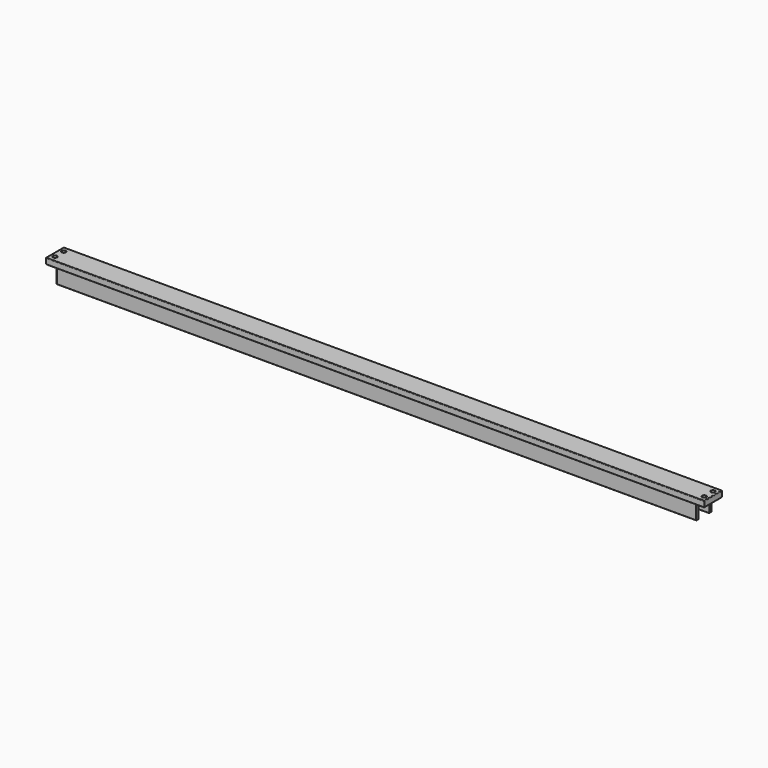
from build123d import *

# Parameters (mm, degrees)
F1_DEPTH = 540
F2_W     = 31
F2_H     = 25
F3_DEPTH = 15
F4_W     = 31
F4_H     = 25
F5_DEPTH = 15
F6_R     = 2
F7_DEPTH = 10.001
F8_R     = 3.5
F9_DEPTH = 4
F10_R    = 1
F11_R    = 1


# Not quite as in the source:
# - a pattern or mirror of a feature is missing from the dataset's text; its kind, count and spacing are read off the source's solid


with BuildPart() as f1:
    # F0 (on Right) → F1 (new body, symmetric)
    with BuildSketch(Plane.YZ):
        Polygon((18.5, 12.5), (-18.5, 12.5), (-18.5, 2.5), (-15.5, 2.5), (-15.5, -22.5), (-10.5, -22.5), (-10.5, 2.5), (0, 2.5), (10.5, 2.5), (10.5, -22.5), (15.5, -22.5), (15.5, 2.5), (18.5, 2.5), align=None)
    extrude(amount=F1_DEPTH, both=True)

    # F2 (on face) → F3 (cut)
    with BuildSketch(Plane(origin=(-540, 0, 0), x_dir=(0, -1, 0), z_dir=(-1, 0, 0))):
        with Locations((0, -10)):
            Rectangle(F2_W, F2_H)
    extrude(amount=-F3_DEPTH, mode=Mode.SUBTRACT)

    # F4 (on face) → F5 (cut)
    with BuildSketch(Plane.YZ.offset(540)):
        with Locations((0, -10)):
            Rectangle(F4_W, F4_H)
    extrude(amount=-F5_DEPTH, mode=Mode.SUBTRACT)

    # F6 (on face) → F7 (cut, through all)
    with BuildSketch(Plane(origin=(0, 0, 2.5), x_dir=(1, 0, 0), z_dir=(0, 0, -1))):
        with Locations((-532.5, 9)):
            Circle(F6_R)
        with Locations((-532.5, -9)):
            Circle(F6_R)
    f7 = extrude(amount=-F7_DEPTH, mode=Mode.SUBTRACT)

    # F7_copies: F7 across plane
    add(f7.mirror(Plane(origin=(0, 0, 0), x_dir=(0, 0, 1), z_dir=(1, 0, 0))), mode=Mode.SUBTRACT)

    # F8 (on face) → F9 (cut)
    with BuildSketch(Plane.XY.offset(12.5)):
        with Locations((-532.5, -9)):
            Circle(F8_R)
        with Locations((-532.5, 9)):
            Circle(F8_R)
    f9 = extrude(amount=-F9_DEPTH, mode=Mode.SUBTRACT)

    # F9_copies: F9 across plane
    add(f9.mirror(Plane(origin=(0, 0, 0), x_dir=(0, 0, 1), z_dir=(1, 0, 0))), mode=Mode.SUBTRACT)

    # F10
    f10_edges = [f1.edges().sort_by_distance(p)[0] for p in [
        (540, 18.5, 7.5),
        (540, -18.5, 7.5),
        (525, 13, -22.5),
        (525, -13, -22.5),
        (-540, -18.5, 7.5),
        (-525, -13, -22.5),
        (-525, 13, -22.5),
        (-540, 18.5, 7.5),
    ]]
    fillet(f10_edges, radius=F10_R)

    # F11
    f11_edges = [f1.edges().sort_by_distance(p)[0] for p in [
        (-525, -10.5, -9.5),
        (-525, -15.5, -9.5),
        (-525, 15.5, -9.5),
        (-525, 10.5, -9.5),
        (-525, 13, -21.5),
        (-525, 13, 2.5),
        (-540, 0, 2.5),
        (-540, 0, 12.5),
        (0, -15.5, 2.5),
        (-539.707107, 18.207107, 12.5),
        (-539.707107, -18.207107, 12.5),
        (0, 18.5, 12.5),
        (0, -18.5, 12.5),
        (539.707107, 18.207107, 12.5),
        (539.707107, -18.207107, 12.5),
        (540, 0, 12.5),
        (-539.707107, 18.207107, 2.5),
        (-539.707107, -18.207107, 2.5),
        (0, 18.5, 2.5),
        (0, -18.5, 2.5),
        (539.707107, 18.207107, 2.5),
        (539.707107, -18.207107, 2.5),
        (540, 0, 2.5),
        (-525, -13, 2.5),
        (525, -13, 2.5),
        (0, -10.5, 2.5),
        (0, 10.5, 2.5),
        (525, 13, 2.5),
        (0, 15.5, 2.5),
        (525, -15.5, -9.5),
        (524.707107, -15.5, -22.207107),
        (0, -15.5, -22.5),
        (-524.707107, -15.5, -22.207107),
        (525, -10.5, -9.5),
        (0, -10.5, -22.5),
        (-524.707107, -10.5, -22.207107),
        (524.707107, -10.5, -22.207107),
        (525, 10.5, -9.5),
        (524.707107, 10.5, -22.207107),
        (0, 10.5, -22.5),
        (-524.707107, 10.5, -22.207107),
        (525, 15.5, -9.5),
        (0, 15.5, -22.5),
        (-524.707107, 15.5, -22.207107),
        (524.707107, 15.5, -22.207107),
    ]]
    fillet(f11_edges, radius=F11_R)


solid = f1.part
